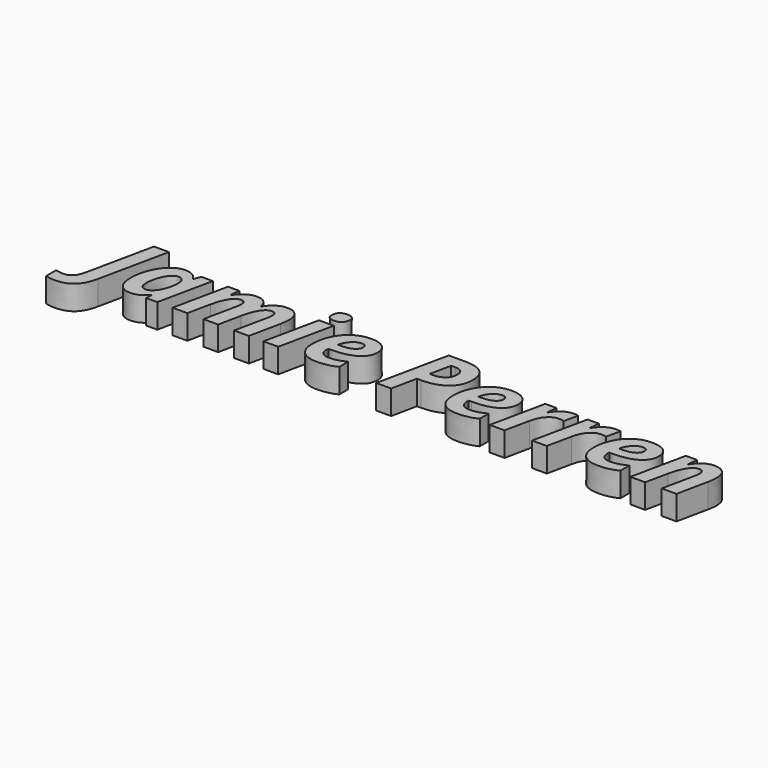
from build123d import *

# Parameters (mm, degrees)
F0_TEXT_SIZE = 105.0505580174
F1_DEPTH     = 25.4


# Not quite as in the source:
# - Text() gives the source's letters only with a copy of the font that has no kerning and outlines rounded to 1/6400 em; it was checked with that copy


with BuildPart() as f1:
    # F0 (on Top) → F1 (new body)
    with BuildSketch(Plane.XY):
        with Locations((-110.8726710081, -8.3507075906)):
            Text('Jamie Perren', F0_TEXT_SIZE, font='Open Sans', font_style=FontStyle.BOLDITALIC, text_align=(TextAlign.LEFT, TextAlign.BOTTOM))
    extrude(amount=F1_DEPTH)


solid = f1.part
